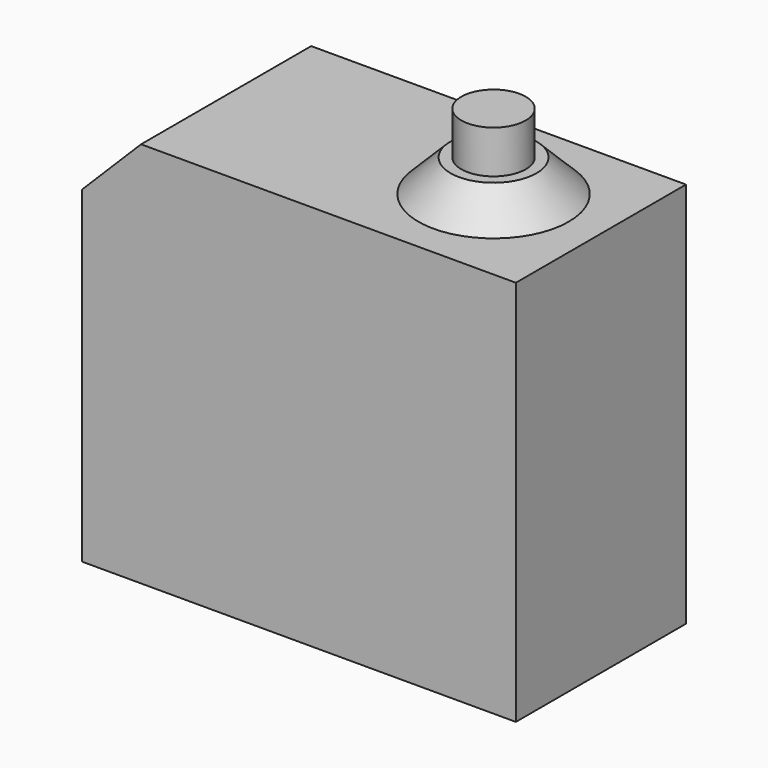
from build123d import *

# Parameters (mm, degrees)
F0_W     = 40.4
F0_H     = 19.8
F1_DEPTH = 36
F2_SIZE  = 5.5
F3_R     = 7
F3_R_2   = 5
F4_DEPTH = 3
F5_DEPTH = 3
F6_SIZE  = 2.99999
F7_R     = 3
F8_DEPTH = 4


# Not quite as in the source:
# - a fillet or chamfer is up to 0.001 mm smaller than in the source, because OpenCascade refuses the exact size


with BuildPart() as f1:
    # F0 (on Top) → F1 (new body)
    with BuildSketch(Plane.XY):
        with Locations((0.6492929533, -3.5976961023)):
            Rectangle(F0_W, F0_H)
    extrude(amount=F1_DEPTH)

    # F2
    f2_edges = [f1.edges().sort_by_distance(p)[0] for p in [
        (-19.550707, -3.597696, 36),
    ]]
    chamfer(f2_edges, length=F2_SIZE)

    # F3 (on face) → F4 (join)
    with BuildSketch(Plane.XY.offset(36)):
        with Locations((10.8492929533, -3.5976961023)):
            Circle(F3_R)
        with Locations((10.8492929533, -3.5976961023)):
            Circle(F3_R_2, mode=Mode.SUBTRACT)
    extrude(amount=F4_DEPTH)

    # F5 (add): a face of the model
    f5_faces = [f1.faces().sort_by_distance(p)[0] for p in [
        (10.8492929533, -3.5976961023, 36),
    ]]
    extrude(f5_faces, amount=F5_DEPTH)

    # F6 (size 3 in the source; OpenCascade refuses exactly that, so slightly less here)
    f6_edges = [f1.edges().sort_by_distance(p)[0] for p in [
        (3.849293, -3.597696, 39),
    ]]
    chamfer(f6_edges, length=F6_SIZE)

    # F7 (on face) → F8 (join)
    with BuildSketch(Plane.XY.offset(39)):
        with Locations((10.8492929533, -3.5976961023)):
            Circle(F7_R)
    extrude(amount=F8_DEPTH)


solid = f1.part
